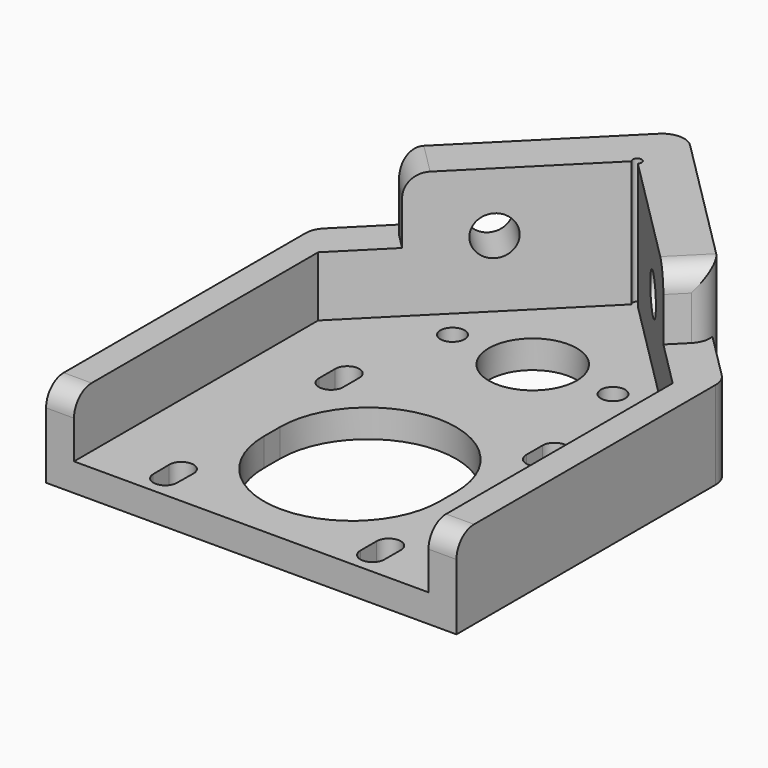
from build123d import *

# Parameters (mm, degrees)
F0_R      = 2.75
F0_R_2    = 10
F1_DEPTH  = 6.35
F3_DEPTH  = 6.35
F4_DEPTH  = 20
F6_DEPTH  = 35
F7_R      = 4.5
F8_DEPTH  = 12.6
F9_R      = 5
F10_R     = 1
F11_DEPTH = 28.65


# Not quite as in the source:
# - a feature names something its author has since deleted; it is built from what else it names


with BuildPart() as f1:
    # F0 (on Top) → F1 (new body)
    with BuildSketch(Plane.XY):
        Polygon((0, 99.6984848098), (-29.6984848098, 70), (-29.6984848098, -10.0008162295), (29.6984848098, -10.0008162295), (29.6984848098, 70), align=None)
        with BuildLine():
            Line((-26.2613506757, -5.0341163975), (-26.3197790794, -0.4248570541))
            ThreePointArc((-26.3197790794, -0.4248570541), (-23.5643542567, 2.3599942046), (-20.8203872227, -0.436147316))
            Line((-20.8203872227, -0.436147316), (-20.892389105, -4.7262623825))
            ThreePointArc((-20.892389105, -4.7262623825), (-23.4159197643, -7.6871530789), (-26.2613506757, -5.0341163975))
        make_face(mode=Mode.SUBTRACT)
        with BuildLine():
            ThreePointArc((-26.32, 46.75), (-23.57, 49.5), (-20.82, 46.75))
            Line((-20.82, 46.75), (-20.82, 42.1391243117))
            ThreePointArc((-20.82, 42.1391243117), (-23.57, 39.3891243117), (-26.32, 42.1391243117))
            Line((-26.32, 42.1391243117), (-26.32, 46.75))
        make_face(mode=Mode.SUBTRACT)
        with BuildLine():
            ThreePointArc((-20, 23.18), (0, 43.18), (20, 23.18))
            Line((20, 23.18), (20, 18.572))
            ThreePointArc((20, 18.572), (0, -1.428), (-20, 18.572))
            Line((-20, 18.572), (-20, 23.18))
        make_face(mode=Mode.SUBTRACT)
        with BuildLine():
            ThreePointArc((20.820000121, -0.3891841763), (23.5802388964, 2.359980939), (26.3199297103, -0.409661849))
            Line((26.3199297103, -0.409661849), (26.290062332, -4.5869490924))
            ThreePointArc((26.290062332, -4.5869490924), (23.7771177689, -7.7443772963), (20.8186322617, -5))
            Line((20.8186322617, -5), (20.820000121, -0.3891841763))
        make_face(mode=Mode.SUBTRACT)
        with BuildLine():
            Line((20.82, 42.1391243117), (20.82, 46.75))
            ThreePointArc((20.82, 46.75), (23.57, 49.5), (26.32, 46.75))
            Line((26.32, 46.75), (26.32, 42.1391243117))
            ThreePointArc((26.32, 42.1391243117), (23.57, 39.3891243117), (20.82, 42.1391243117))
        make_face(mode=Mode.SUBTRACT)
        with Locations((-18.25, 70)):
            Circle(F0_R, mode=Mode.SUBTRACT)
        with Locations((0, 70)):
            Circle(F0_R_2, mode=Mode.SUBTRACT)
        with Locations((18.25, 70)):
            Circle(F0_R, mode=Mode.SUBTRACT)
    extrude(amount=F1_DEPTH)

    # F2 (on Top) → F3 (join)
    with BuildSketch(Plane.XY):
        Polygon((-29.6984848098, 70), (0, 99.6984848098), (0, 112.4264068712), (-46.6550865276, 65.7713203436), (-46.6550865276, 53.0433982822), (-40.3050865276, 59.3933982822), align=None)
        Polygon((-29.6984848098, -10.0008162295), (-29.6984848098, 70), (-40.3050865276, 59.3933982822), (-40.3050865276, -10.0008162295), align=None)
        Polygon((-40.3050865276, -10.0008162295), (-40.3050865276, 59.3933982822), (-46.6550865276, 53.0433982822), (-46.6550865276, -10.0008162295), align=None)
        Polygon((40.3050865276, 59.3933982822), (29.6984848098, 70), (29.6984848098, -10.0008162295), (40.3050865276, -10.0008162295), align=None)
        Polygon((46.6550865276, 53.0433982822), (40.3050865276, 59.3933982822), (40.3050865276, -10.0008162295), (46.6550865276, -10.0008162295), align=None)
        Polygon((0, 112.4264068712), (0, 99.6984848098), (29.6984848098, 70), (40.3050865276, 59.3933982822), (46.6550865276, 53.0433982822), (46.6550865276, 65.7713203436), align=None)
    extrude(amount=F3_DEPTH)

    # F2 (on Top) → F4 (join)
    with BuildSketch(Plane.XY):
        Polygon((46.6550865276, 53.0433982822), (40.3050865276, 59.3933982822), (40.3050865276, -10.0008162295), (46.6550865276, -10.0008162295), align=None)
        Polygon((-40.3050865276, -10.0008162295), (-40.3050865276, 59.3933982822), (-46.6550865276, 53.0433982822), (-46.6550865276, -10.0008162295), align=None)
        Polygon((0, 112.4264068712), (0, 99.6984848098), (29.6984848098, 70), (40.3050865276, 59.3933982822), (46.6550865276, 53.0433982822), (46.6550865276, 65.7713203436), align=None)
        Polygon((-29.6984848098, 70), (0, 99.6984848098), (0, 112.4264068712), (-46.6550865276, 65.7713203436), (-46.6550865276, 53.0433982822), (-40.3050865276, 59.3933982822), align=None)
    extrude(amount=F4_DEPTH)

    # F5 (on face) → F6 (join)
    with BuildSketch(Plane(origin=(0, 0, 0), x_dir=(1, 0, 0), z_dir=(0, 0, -1))):
        Polygon((0, -99.6984848098), (-29.6984848098, -70), (-36.7695526217, -77.0710678119), (-5.8406204336, -108), (0, -113.8406204336), (5.8406204336, -108), (36.7695526217, -77.0710678119), (29.6984848098, -70), align=None)
    extrude(amount=-F6_DEPTH)

    # F9 (call 1 of 7: OpenCascade refuses the feature's edges together)
    f9_edges = [f1.edges().sort_by_distance(p)[0] for p in [
        (33.234019, 73.535534, 35),
        (36.769553, 77.071068, 17.5),
    ]]
    fillet(f9_edges, radius=F9_R)

    # F9#2 (call 2 of 7)
    f9_2_edges = [f1.edges().sort_by_distance(p)[0] for p in [
        (-33.234019, 73.535534, 35),
        (-36.769553, 77.071068, 17.5),
    ]]
    fillet(f9_2_edges, radius=F9_R)

    # F9#3 (call 3 of 7)
    f9_3_edges = [f1.edges().sort_by_distance(p)[0] for p in [
        (43.480087, -10.000816, 20),
    ]]
    fillet(f9_3_edges, radius=F9_R)

    # F9#4 (call 4 of 7)
    f9_4_edges = [f1.edges().sort_by_distance(p)[0] for p in [
        (-43.480087, -10.000816, 20),
    ]]
    fillet(f9_4_edges, radius=F9_R)

    # F9#5 (call 5 of 7)
    f9_5_edges = [f1.edges().sort_by_distance(p)[0] for p in [
        (46.655087, 65.77132, 10),
    ]]
    fillet(f9_5_edges, radius=F9_R)

    # F9#6 (call 6 of 7)
    f9_6_edges = [f1.edges().sort_by_distance(p)[0] for p in [
        (0, 113.84062, 17.5),
    ]]
    fillet(f9_6_edges, radius=F9_R)

    # F9#7 (call 7 of 7)
    f9_7_edges = [f1.edges().sort_by_distance(p)[0] for p in [
        (-46.655087, 65.77132, 10),
    ]]
    fillet(f9_7_edges, radius=F9_R)

    # F10 (on face) → F11 (cut, through all)
    with BuildSketch(Plane.XY.offset(35)):
        with Locations((0, 99.6984848098)):
            Circle(F10_R)
    extrude(amount=-F11_DEPTH, mode=Mode.SUBTRACT)


with BuildPart() as f8:
    # F7 (on face) → F8 (new body)
    with BuildSketch(Plane(origin=(56.9203102168, 56.9203102168, 0), x_dir=(-0.7071067812, 0.7071067812, 0), z_dir=(0.7071067812, 0.7071067812, 0))):
        with Locations((44.9974746831, 21.5)):
            Circle(F7_R)
    extrude(amount=-F8_DEPTH)


with BuildPart() as f12_1:
    # F12: instance of F8
    add(f8.part.mirror(Plane.YZ))


with BuildPart() as f1_1:
    add(f1.part)

    # F13: cut F12_1, F8
    add(f12_1.part, mode=Mode.SUBTRACT)
    add(f8.part, mode=Mode.SUBTRACT)


solid = f1_1.part
